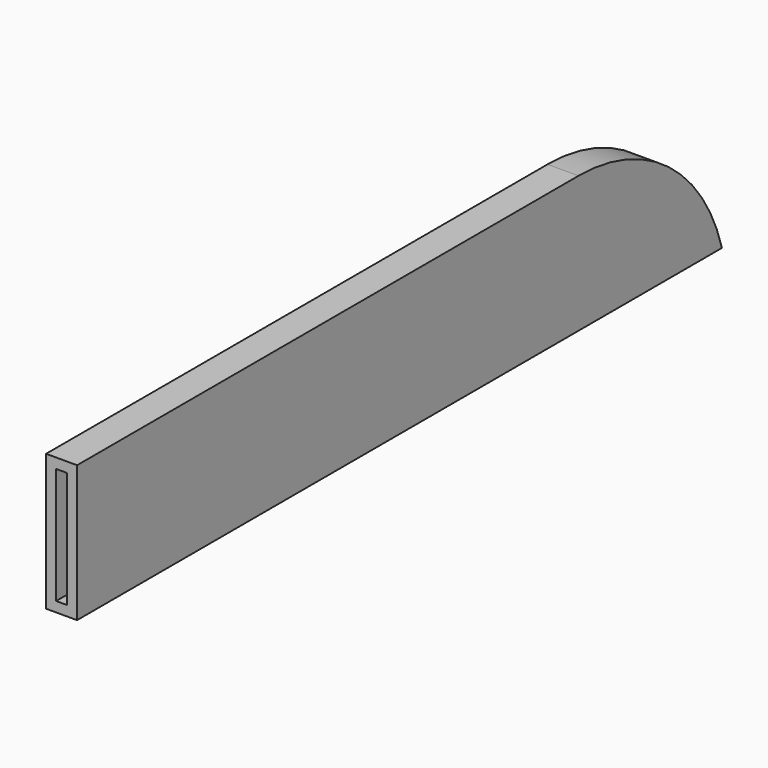
from build123d import *

# Parameters (mm, degrees)
F0_W        = 130
F0_H        = 22
F1_DEPTH    = 5
F2_T1_DEPTH = 149.568322948
F3_T        = -1.625


# Not quite as in the source:
# - a fillet or chamfer that OpenCascade refuses, or shapes differently, is made with other operations: its cross-section is extruded or revolved along the edge and cut away or added


with BuildPart() as f1:
    # F0 (on Right) → F1 (new body)
    with BuildSketch(Plane.YZ):
        with Locations((-0.3712646805, 30.1455706358)):
            Rectangle(F0_W, F0_H)
    extrude(amount=F1_DEPTH)

    # F2: fillet of radius 30 on 1 edges, made by hand

    # F2_s2 → F2_t1 (cut)
    with BuildSketch(Plane.YZ.offset(-72.284161474)):
        with BuildLine():
            ThreePointArc((35.7150707299, 41.1455706358), (53.8809728545, 35.0202434084), (64.6287353195, 19.1455706358))
            Line((64.6287353195, 19.1455706358), (64.6287353195, 41.1455706358))
            Line((64.6287353195, 41.1455706358), (35.7150707299, 41.1455706358))
        make_face()
    extrude(amount=F2_T1_DEPTH, mode=Mode.SUBTRACT)

    # F3
    f3_openings = [f1.faces().sort_by_distance(p)[0] for p in [
        (2.5, -65.371265, 30.145571),
    ]]
    offset(amount=F3_T, openings=f3_openings)


solid = f1.part
